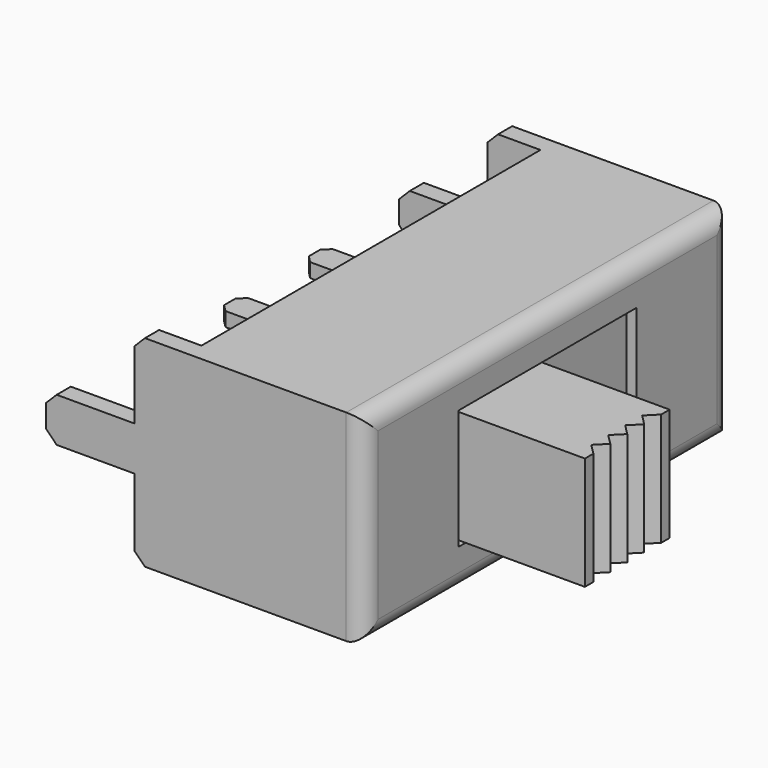
from build123d import *

# Parameters (mm, degrees)
F0_W       = 5
F0_H       = 13
F1_DEPTH   = 5.7
F2_W       = 6.3
F2_H       = 3.4
F3_DEPTH   = 2
F4_W       = 6.1
F4_H       = 3.2
F5_DEPTH   = 1.8
F6_W       = 3
F6_H       = 3.2
F7_DEPTH   = 3.7
F8_W       = 0.5
F8_H       = 5.7
F9_DEPTH   = 1.5
F10_R      = 0.5
F11_W      = 11.6
F11_H      = 5.3
F12_DEPTH  = 2
F13_W      = 0.5
F13_H      = 11
F14_DEPTH  = 5.3
F17_DEPTH  = 25
F15_W      = 2
F15_H      = 0.4
F18_DEPTH  = 0.5
F19_W      = 0.8
F19_H      = 0.4
F22_DEPTH  = 3.5
F20_W      = 0.8
F20_H      = 0.4
F21_W      = 0.8
F21_H      = 0.4
F23_W      = 0.5
F23_H      = 1.25
F24_W      = 0.5
F24_H      = 1.25
F25_DEPTH  = 2.5
F26_SIZE   = 0.2
F26_2_SIZE = 0.2
F26_3_SIZE = 0.2
F27_SIZE   = 0.3
F28_SIZE   = 0.3


with BuildPart() as f1:
    # F0 (on Top) → F1 (new body)
    with BuildSketch(Plane.XY):
        Rectangle(F0_W, F0_H)
    extrude(amount=F1_DEPTH)

    # F2 (on face) → F3 (cut)
    with BuildSketch(Plane.YZ.offset(2.5)):
        with Locations((0, 2.85)):
            Rectangle(F2_W, F2_H)
    extrude(amount=-F3_DEPTH, mode=Mode.SUBTRACT)

    # F8 (on face) → F9 (join)
    with BuildSketch(Plane(origin=(-2.5, 0, 0), x_dir=(0, -1, 0), z_dir=(-1, 0, 0))):
        with Locations((-6.25, 2.85)):
            Rectangle(F8_W, F8_H)
        with Locations((6.25, 2.85)):
            Rectangle(F8_W, F8_H)
    extrude(amount=F9_DEPTH)

    # F10
    f10_edges = [f1.edges().sort_by_distance(p)[0] for p in [
        (2.5, 0, 5.7),
        (2.5, 6.5, 2.85),
        (2.5, 0, 0),
        (2.5, -6.5, 2.85),
    ]]
    fillet(f10_edges, radius=F10_R)

    # F11 (on face) → F12 (cut)
    with BuildSketch(Plane(origin=(-2.5, 0, 0), x_dir=(0, -1, 0), z_dir=(-1, 0, 0))):
        with Locations((0, 2.85)):
            Rectangle(F11_W, F11_H)
    extrude(amount=-F12_DEPTH, mode=Mode.SUBTRACT)

    # F23 (on face) + F24 (on face) → F25 (join)
    with BuildSketch(Plane(origin=(-4, 0, 0), x_dir=(0, -1, 0), z_dir=(-1, 0, 0))):
        with Locations((-6.25, 2.85)):
            Rectangle(F23_W, F23_H)
    with BuildSketch(Plane(origin=(-4, 0, 0), x_dir=(0, -1, 0), z_dir=(-1, 0, 0))):
        with Locations((6.25, 2.85)):
            Rectangle(F24_W, F24_H)
    extrude(amount=F25_DEPTH)

    # F27
    f27_edges = [f1.edges().sort_by_distance(p)[0] for p in [
        (-6.5, -6.25, 3.475),
        (-6.5, -6.25, 2.225),
        (-6.5, 6.25, 3.475),
        (-6.5, 6.25, 2.225),
    ]]
    chamfer(f27_edges, length=F27_SIZE)

    # F28
    f28_edges = [f1.edges().sort_by_distance(p)[0] for p in [
        (-4, 6.25, 5.7),
        (-4, 6.25, 0),
        (-4, -6.25, 5.7),
        (-4, -6.25, 0),
    ]]
    chamfer(f28_edges, length=F28_SIZE)


with BuildPart() as f5:
    # F4 (on face) → F5 (new body)
    with BuildSketch(Plane.YZ.offset(0.5)):
        with Locations((0, 2.85)):
            Rectangle(F4_W, F4_H)
    extrude(amount=F5_DEPTH)

    # F6 (on face) → F7 (join)
    with BuildSketch(Plane.YZ.offset(2.3)):
        with Locations((-1.55, 2.85)):
            Rectangle(F6_W, F6_H)
    extrude(amount=F7_DEPTH)

    # F16 (on face) → F17 (cut)
    with BuildSketch(Plane(origin=(0, 0, 1.25), x_dir=(1, 0, 0), z_dir=(0, 0, -1))):
        Polygon((6, 2.15), (6, 2.75), (5.7, 2.45), align=None)
        Polygon((6, 1.55), (6, 2.15), (5.7, 1.85), align=None)
        Polygon((6, 0.95), (6, 1.55), (5.7, 1.25), align=None)
        Polygon((6, 0.35), (6, 0.95), (5.7, 0.65), align=None)
    extrude(amount=-F17_DEPTH, mode=Mode.SUBTRACT)


with BuildPart() as f14:
    # F13 (on face) → F14 (new body)
    with BuildSketch(Plane(origin=(0, 0, 5.5), x_dir=(1, 0, 0), z_dir=(0, 0, -1))):
        with Locations((-2.25, 0)):
            Rectangle(F13_W, F13_H)
    extrude(amount=F14_DEPTH)


with BuildPart() as f18:
    # F15 (on face) → F18 (new body)
    with BuildSketch(Plane(origin=(-2.5, 0, 0), x_dir=(0, -1, 0), z_dir=(-1, 0, 0))):
        with Locations((-3, 2.85)):
            Rectangle(F15_W, F15_H)
    extrude(amount=F18_DEPTH)


with BuildPart() as f18b:
    # F15 (on face) → F18, piece 2 (new body)
    with BuildSketch(Plane(origin=(-2.5, 0, 0), x_dir=(0, -1, 0), z_dir=(-1, 0, 0))):
        with Locations((0, 2.85)):
            Rectangle(F15_W, F15_H)
    extrude(amount=F18_DEPTH)


with BuildPart() as f18c:
    # F15 (on face) → F18, piece 3 (new body)
    with BuildSketch(Plane(origin=(-2.5, 0, 0), x_dir=(0, -1, 0), z_dir=(-1, 0, 0))):
        with Locations((3, 2.85)):
            Rectangle(F15_W, F15_H)
    extrude(amount=F18_DEPTH)


with BuildPart() as f22:
    # F19 (on face) → F22 (new body)
    with BuildSketch(Plane(origin=(-3, 0, 0), x_dir=(0, -1, 0), z_dir=(-1, 0, 0))):
        with Locations((-3, 2.85)):
            Rectangle(F19_W, F19_H)
    extrude(amount=F22_DEPTH)

    # F26
    f26_edges = [f22.edges().sort_by_distance(p)[0] for p in [
        (-6.5, 3.4, 2.85),
        (-6.5, 2.6, 2.85),
    ]]
    chamfer(f26_edges, length=F26_SIZE)


with BuildPart() as f22b:
    # F20 (on face) → F22, piece 2 (new body)
    with BuildSketch(Plane(origin=(-3, 0, 0), x_dir=(0, -1, 0), z_dir=(-1, 0, 0))):
        with Locations((0, 2.85)):
            Rectangle(F20_W, F20_H)
    extrude(amount=F22_DEPTH)

    # F26#2
    f26_2_edges = [f22b.edges().sort_by_distance(p)[0] for p in [
        (-6.5, 0.4, 2.85),
        (-6.5, -0.4, 2.85),
    ]]
    chamfer(f26_2_edges, length=F26_2_SIZE)


with BuildPart() as f22c:
    # F21 (on face) → F22, piece 3 (new body)
    with BuildSketch(Plane(origin=(-3, 0, 0), x_dir=(0, -1, 0), z_dir=(-1, 0, 0))):
        with Locations((3, 2.85)):
            Rectangle(F21_W, F21_H)
    extrude(amount=F22_DEPTH)

    # F26#3
    f26_3_edges = [f22c.edges().sort_by_distance(p)[0] for p in [
        (-6.5, -2.6, 2.85),
        (-6.5, -3.4, 2.85),
    ]]
    chamfer(f26_3_edges, length=F26_3_SIZE)


solid = Compound([f1.part, f5.part, f14.part, f18.part, f18b.part, f18c.part, f22.part, f22b.part, f22c.part])
